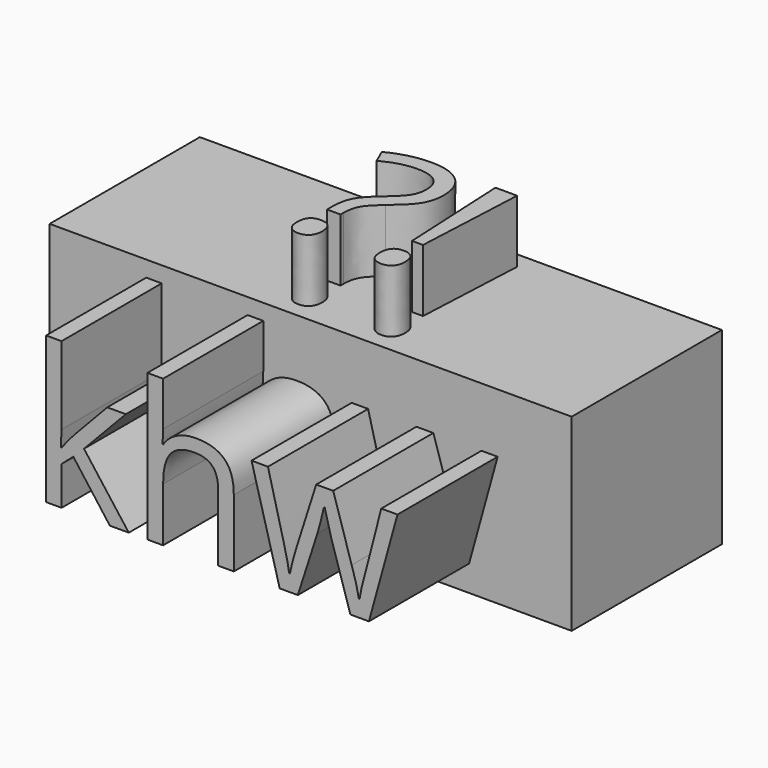
from build123d import *

# Parameters (mm, degrees)
F0_W         = 105.9118509293
F0_H         = 38.2536314428
F1_DEPTH     = 38.1
F2_TEXT_SIZE = 39.1754011313
F3_DEPTH     = 25.4
F4_TEXT_SIZE = 43.5282246649
F5_DEPTH     = 12.7


# Not quite as in the source:
# - Text() gives the source's letters only with a copy of the font that has no kerning and outlines rounded to 1/6400 em; it was checked with that copy


with BuildPart() as f1:
    # F0 (on Front) → F1 (new body)
    with BuildSketch(Plane.XZ):
        with Locations((52.9559254646, 19.1268157214)):
            Rectangle(F0_W, F0_H)
    extrude(amount=F1_DEPTH)

    # F2 (on face) → F3 (join)
    with BuildSketch(Plane.XZ.offset(38.1)):
        with Locations((16.2385841832, 5.2541159093)):
            Text('khw', F2_TEXT_SIZE, font='Open Sans', text_align=(TextAlign.LEFT, TextAlign.BOTTOM))
    extrude(amount=F3_DEPTH)

    # F4 (on face) → F5 (join)
    with BuildSketch(Plane.XY.offset(38.2536314428)):
        with Locations((40.3441861272, -34.4192925841)):
            Text('?!', F4_TEXT_SIZE, font='Open Sans', text_align=(TextAlign.LEFT, TextAlign.BOTTOM))
    extrude(amount=F5_DEPTH)


solid = f1.part
